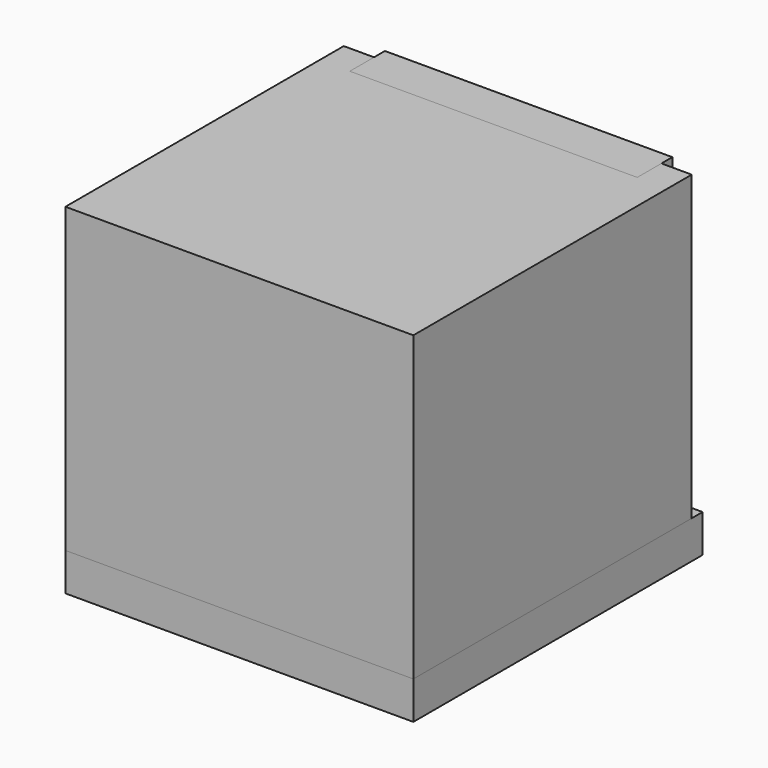
from build123d import *

# Parameters (mm, degrees)
F1_R     = 2
F2_DEPTH = 5
F3_DEPTH = 10
F4_DEPTH = 45
F5_START = 5
F5_DEPTH = 40
F6_START = 40
F6_DEPTH = 5
F7_W     = 20
F7_H     = 32
F8_DEPTH = 1.8


with BuildPart() as f2:
    # F1 (on Top) → F2 (new body)
    with BuildSketch(Plane.XY):
        with BuildLine():
            Line((110, 142), (104, 142))
            Line((104, 142), (104, 136))
            Line((104, 136), (107, 136))
            ThreePointArc((107, 136), (109.1213203436, 136.8786796564), (110, 139))
            Line((110, 139), (110, 142))
        make_face()
        with Locations((107, 139)):
            Circle(F1_R, mode=Mode.SUBTRACT)
        with BuildLine():
            Line((136, 142), (110, 142))
            Line((110, 142), (110, 139))
            ThreePointArc((110, 139), (109.1213203436, 136.8786796564), (107, 136))
            Line((107, 136), (104, 136))
            Line((104, 136), (104, 110))
            Line((104, 110), (107, 110))
            ThreePointArc((107, 110), (109.1213203436, 109.1213203436), (110, 107))
            Line((110, 107), (110, 104))
            Line((110, 104), (136, 104))
            Line((136, 104), (136, 107))
            ThreePointArc((136, 107), (136.8786796564, 109.1213203436), (139, 110))
            Line((139, 110), (142, 110))
            Line((142, 110), (142, 136))
            Line((142, 136), (139, 136))
            ThreePointArc((139, 136), (136.8786796564, 136.8786796564), (136, 139))
            Line((136, 139), (136, 142))
        make_face()
        Polygon((100, 146), (100, 100), (146, 100), (146, 146), (142, 146), (142, 142), (142, 136), (142, 110), (142, 104), (136, 104), (110, 104), (104, 104), (104, 110), (104, 136), (104, 142), (104, 146), align=None)
        with BuildLine():
            Line((142, 136), (142, 142))
            Line((142, 142), (136, 142))
            Line((136, 142), (136, 139))
            ThreePointArc((136, 139), (136.8786796564, 136.8786796564), (139, 136))
            Line((139, 136), (142, 136))
        make_face()
        with Locations((139, 139)):
            Circle(F1_R, mode=Mode.SUBTRACT)
        with BuildLine():
            Line((107, 110), (104, 110))
            Line((104, 110), (104, 104))
            Line((104, 104), (110, 104))
            Line((110, 104), (110, 107))
            ThreePointArc((110, 107), (109.1213203436, 109.1213203436), (107, 110))
        make_face()
        with Locations((107, 107)):
            Circle(F1_R, mode=Mode.SUBTRACT)
        with BuildLine():
            Line((142, 104), (142, 110))
            Line((142, 110), (139, 110))
            ThreePointArc((139, 110), (136.8786796564, 109.1213203436), (136, 107))
            Line((136, 107), (136, 104))
            Line((136, 104), (142, 104))
        make_face()
        with Locations((139, 107)):
            Circle(F1_R, mode=Mode.SUBTRACT)
        Polygon((142, 146), (104, 146), (104, 142), (110, 142), (136, 142), (142, 142), align=None)
    extrude(amount=F2_DEPTH)

    # F1 (on Top) → F3 (join)
    with BuildSketch(Plane.XY):
        with BuildLine():
            Line((110, 142), (104, 142))
            Line((104, 142), (104, 136))
            Line((104, 136), (107, 136))
            ThreePointArc((107, 136), (109.1213203436, 136.8786796564), (110, 139))
            Line((110, 139), (110, 142))
        make_face()
        with Locations((107, 139)):
            Circle(F1_R, mode=Mode.SUBTRACT)
        with BuildLine():
            Line((142, 136), (142, 142))
            Line((142, 142), (136, 142))
            Line((136, 142), (136, 139))
            ThreePointArc((136, 139), (136.8786796564, 136.8786796564), (139, 136))
            Line((139, 136), (142, 136))
        make_face()
        with Locations((139, 139)):
            Circle(F1_R, mode=Mode.SUBTRACT)
        with BuildLine():
            Line((107, 110), (104, 110))
            Line((104, 110), (104, 104))
            Line((104, 104), (110, 104))
            Line((110, 104), (110, 107))
            ThreePointArc((110, 107), (109.1213203436, 109.1213203436), (107, 110))
        make_face()
        with Locations((107, 107)):
            Circle(F1_R, mode=Mode.SUBTRACT)
        with BuildLine():
            Line((142, 104), (142, 110))
            Line((142, 110), (139, 110))
            ThreePointArc((139, 110), (136.8786796564, 109.1213203436), (136, 107))
            Line((136, 107), (136, 104))
            Line((136, 104), (142, 104))
        make_face()
        with Locations((139, 107)):
            Circle(F1_R, mode=Mode.SUBTRACT)
    extrude(amount=F3_DEPTH)

    # F1 (on Top) → F4 (join)
    with BuildSketch(Plane.XY):
        Polygon((142, 146), (104, 146), (104, 142), (110, 142), (136, 142), (142, 142), align=None)
    extrude(amount=F4_DEPTH)

    # F7 (on face) → F8 (join)
    with BuildSketch(Plane(origin=(0, 146, 0), x_dir=(-1, 0, 0), z_dir=(0, 1, 0))):
        Polygon((-146, 5), (-146, 0), (-100, 0), (-100, 5), (-104, 5), (-104, 45), (-142, 45), (-142, 5), align=None)
        with Locations((-123, 25)):
            Rectangle(F7_W, F7_H, mode=Mode.SUBTRACT)
    extrude(amount=F8_DEPTH)


with BuildPart() as f5:
    # F1 (on Top) → F5 (new body)
    with BuildSketch(Plane.XY.offset(F5_START)):
        Polygon((100, 146), (100, 100), (146, 100), (146, 146), (142, 146), (142, 142), (142, 136), (142, 110), (142, 104), (136, 104), (110, 104), (104, 104), (104, 110), (104, 136), (104, 142), (104, 146), align=None)
    extrude(amount=F5_DEPTH)

    # F1 (on Top) → F6 (join)
    with BuildSketch(Plane.XY.offset(F6_START)):
        with BuildLine():
            Line((136, 142), (110, 142))
            Line((110, 142), (110, 139))
            ThreePointArc((110, 139), (109.1213203436, 136.8786796564), (107, 136))
            Line((107, 136), (104, 136))
            Line((104, 136), (104, 110))
            Line((104, 110), (107, 110))
            ThreePointArc((107, 110), (109.1213203436, 109.1213203436), (110, 107))
            Line((110, 107), (110, 104))
            Line((110, 104), (136, 104))
            Line((136, 104), (136, 107))
            ThreePointArc((136, 107), (136.8786796564, 109.1213203436), (139, 110))
            Line((139, 110), (142, 110))
            Line((142, 110), (142, 136))
            Line((142, 136), (139, 136))
            ThreePointArc((139, 136), (136.8786796564, 136.8786796564), (136, 139))
            Line((136, 139), (136, 142))
        make_face()
        with BuildLine():
            Line((107, 110), (104, 110))
            Line((104, 110), (104, 104))
            Line((104, 104), (110, 104))
            Line((110, 104), (110, 107))
            ThreePointArc((110, 107), (109.1213203436, 109.1213203436), (107, 110))
        make_face()
        with Locations((107, 107)):
            Circle(F1_R, mode=Mode.SUBTRACT)
        with BuildLine():
            Line((142, 104), (142, 110))
            Line((142, 110), (139, 110))
            ThreePointArc((139, 110), (136.8786796564, 109.1213203436), (136, 107))
            Line((136, 107), (136, 104))
            Line((136, 104), (142, 104))
        make_face()
        with Locations((139, 107)):
            Circle(F1_R, mode=Mode.SUBTRACT)
        with BuildLine():
            Line((142, 136), (142, 142))
            Line((142, 142), (136, 142))
            Line((136, 142), (136, 139))
            ThreePointArc((136, 139), (136.8786796564, 136.8786796564), (139, 136))
            Line((139, 136), (142, 136))
        make_face()
        with Locations((139, 139)):
            Circle(F1_R, mode=Mode.SUBTRACT)
        with BuildLine():
            Line((110, 142), (104, 142))
            Line((104, 142), (104, 136))
            Line((104, 136), (107, 136))
            ThreePointArc((107, 136), (109.1213203436, 136.8786796564), (110, 139))
            Line((110, 139), (110, 142))
        make_face()
        with Locations((107, 139)):
            Circle(F1_R, mode=Mode.SUBTRACT)
        with Locations((107, 107)):
            Circle(F1_R)
        with Locations((139, 107)):
            Circle(F1_R)
        with Locations((107, 139)):
            Circle(F1_R)
        with Locations((139, 139)):
            Circle(F1_R)
    extrude(amount=F6_DEPTH)


solid = Compound([f2.part, f5.part])
